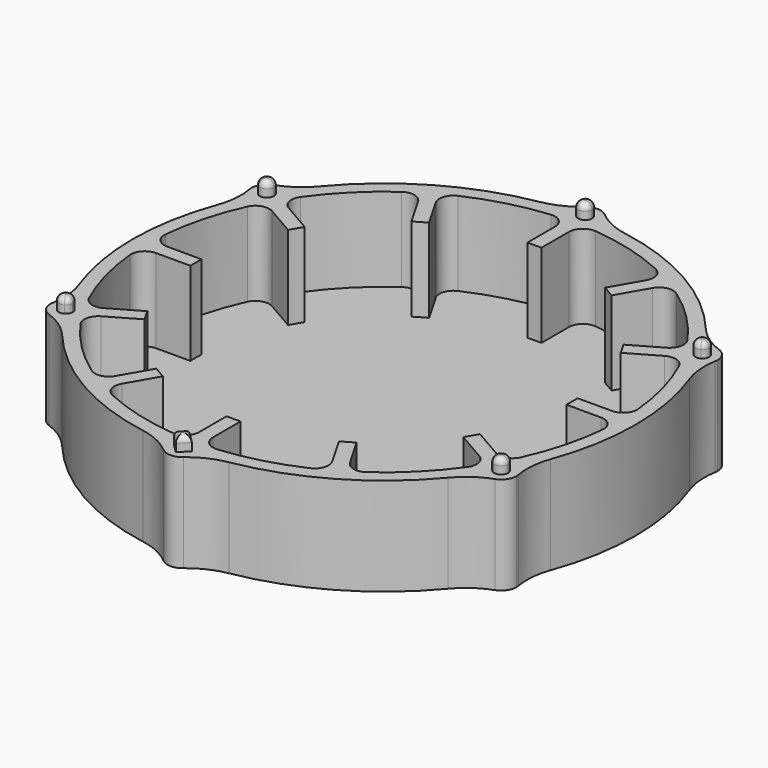
from build123d import *

# Parameters (mm, degrees)
F1_R      = 18
F1_R_2    = 17
F2_DEPTH  = 7
F3_DEPTH  = 7
F4_DEPTH  = 1
F6_DEPTH  = 7
F7_R      = 1
F8_R      = 5
F9_DEPTH  = 8
F10_R     = 0.44999
F11_DEPTH = 1.8


# Not quite as in the source:
# - a fillet or chamfer is up to 0.001 mm smaller than in the source, because OpenCascade refuses the exact size


with BuildPart() as f2:
    # F1 (on Top) → F2 (new body)
    with BuildSketch(Plane.XY):
        Circle(F1_R)
        Circle(F1_R_2, mode=Mode.SUBTRACT)
    extrude(amount=F2_DEPTH)

    # F0 (on Top) → F3 (join)
    with BuildSketch(Plane.XY):
        with BuildLine():
            Line((-11.4073228059, 7.1633711619), (-14.4660626528, 8.9293354359))
            ThreePointArc((-14.4660626528, 8.9293354359), (-14.7224318643, 8.5), (-14.9660626528, 8.0633100321))
            Line((-14.9660626528, 8.0633100321), (-11.9073228059, 6.2973457581))
            ThreePointArc((-11.9073228059, 6.2973457581), (-11.665362189, 6.735), (-11.4073228059, 7.1633711619))
        make_face()
        with BuildLine():
            Line((7.1633711619, 11.4073228059), (8.9293354359, 14.4660626528))
            ThreePointArc((8.9293354359, 14.4660626528), (8.5, 14.7224318643), (8.0633100321, 14.9660626528))
            Line((8.0633100321, 14.9660626528), (6.2973457581, 11.9073228059))
            ThreePointArc((6.2973457581, 11.9073228059), (6.735, 11.665362189), (7.1633711619, 11.4073228059))
        make_face()
        with BuildLine():
            ThreePointArc((17, 0), (16.9981612676, 0.2500270431), (16.992645468, 0.5))
            Line((16.992645468, 0.5), (13.46071692, 0.5))
            ThreePointArc((13.46071692, 0.5), (13.46767903, 0.2500430841), (13.47, 0))
            ThreePointArc((13.47, 0), (13.46767903, -0.2500430841), (13.46071692, -0.5))
            Line((13.46071692, -0.5), (16.992645468, -0.5))
            ThreePointArc((16.992645468, -0.5), (16.9981612676, -0.2500270431), (17, 0))
        make_face()
        with BuildLine():
            ThreePointArc((-0.5, -16.992645468), (0, -17), (0.5, -16.992645468))
            Line((0.5, -16.992645468), (0.5, -13.46071692))
            ThreePointArc((0.5, -13.46071692), (0, -13.47), (-0.5, -13.46071692))
            Line((-0.5, -13.46071692), (-0.5, -16.992645468))
        make_face()
        with BuildLine():
            ThreePointArc((-14.9660626528, -8.0633100321), (-14.7224318643, -8.5), (-14.4660626528, -8.9293354359))
            Line((-14.4660626528, -8.9293354359), (-11.4073228059, -7.1633711619))
            ThreePointArc((-11.4073228059, -7.1633711619), (-11.665362189, -6.735), (-11.9073228059, -6.2973457581))
            Line((-11.9073228059, -6.2973457581), (-14.9660626528, -8.0633100321))
        make_face()
        with BuildLine():
            Line((-6.2973457581, 11.9073228059), (-8.0633100321, 14.9660626528))
            ThreePointArc((-8.0633100321, 14.9660626528), (-8.5, 14.7224318643), (-8.9293354359, 14.4660626528))
            Line((-8.9293354359, 14.4660626528), (-7.1633711619, 11.4073228059))
            ThreePointArc((-7.1633711619, 11.4073228059), (-6.735, 11.665362189), (-6.2973457581, 11.9073228059))
        make_face()
        with BuildLine():
            Line((0.5, 13.46071692), (0.5, 16.992645468))
            ThreePointArc((0.5, 16.992645468), (0, 17), (-0.5, 16.992645468))
            Line((-0.5, 16.992645468), (-0.5, 13.46071692))
            ThreePointArc((-0.5, 13.46071692), (0, 13.47), (0.5, 13.46071692))
        make_face()
        with BuildLine():
            Line((11.9073228059, 6.2973457581), (14.9660626528, 8.0633100321))
            ThreePointArc((14.9660626528, 8.0633100321), (14.7224318643, 8.5), (14.4660626528, 8.9293354359))
            Line((14.4660626528, 8.9293354359), (11.4073228059, 7.1633711619))
            ThreePointArc((11.4073228059, 7.1633711619), (11.665362189, 6.735), (11.9073228059, 6.2973457581))
        make_face()
        with BuildLine():
            ThreePointArc((14.4660626528, -8.9293354359), (14.7224318643, -8.5), (14.9660626528, -8.0633100321))
            Line((14.9660626528, -8.0633100321), (11.9073228059, -6.2973457581))
            ThreePointArc((11.9073228059, -6.2973457581), (11.665362189, -6.735), (11.4073228059, -7.1633711619))
            Line((11.4073228059, -7.1633711619), (14.4660626528, -8.9293354359))
        make_face()
        with BuildLine():
            ThreePointArc((8.0633100321, -14.9660626528), (8.5, -14.7224318643), (8.9293354359, -14.4660626528))
            Line((8.9293354359, -14.4660626528), (7.1633711619, -11.4073228059))
            ThreePointArc((7.1633711619, -11.4073228059), (6.735, -11.665362189), (6.2973457581, -11.9073228059))
            Line((6.2973457581, -11.9073228059), (8.0633100321, -14.9660626528))
        make_face()
        with BuildLine():
            ThreePointArc((-8.9293354359, -14.4660626528), (-8.5, -14.7224318643), (-8.0633100321, -14.9660626528))
            Line((-8.0633100321, -14.9660626528), (-6.2973457581, -11.9073228059))
            ThreePointArc((-6.2973457581, -11.9073228059), (-6.735, -11.665362189), (-7.1633711619, -11.4073228059))
            Line((-7.1633711619, -11.4073228059), (-8.9293354359, -14.4660626528))
        make_face()
        with BuildLine():
            Line((-13.46071692, 0.5), (-16.992645468, 0.5))
            ThreePointArc((-16.992645468, 0.5), (-17, 0), (-16.992645468, -0.5))
            Line((-16.992645468, -0.5), (-13.46071692, -0.5))
            ThreePointArc((-13.46071692, -0.5), (-13.47, 0), (-13.46071692, 0.5))
        make_face()
    extrude(amount=F3_DEPTH)

    # F1 (on Top) → F4 (join)
    with BuildSketch(Plane.XY):
        Circle(F1_R)
        Circle(F1_R_2, mode=Mode.SUBTRACT)
        Circle(F1_R_2)
    extrude(amount=F4_DEPTH)

    # F5 (on Top) → F6 (join)
    with BuildSketch(Plane.XY):
        with BuildLine():
            ThreePointArc((-14.4884572681, 9), (-14.6275367743, 9.5353800561), (-15.0096060035, 9.935377578))
            ThreePointArc((-15.0096060035, 9.935377578), (-15.1731450826, 9.6837837802), (-15.3324673166, 9.4294987133))
            ThreePointArc((-15.3324673166, 9.4294987133), (-15.153718855, 9.2469868663), (-15.0884572681, 9))
            ThreePointArc((-15.0884572681, 9), (-15.3354561915, 8.5687338928), (-15.832419089, 8.5635568422))
            ThreePointArc((-15.832419089, 8.5635568422), (-15.9729752997, 8.2984372068), (-16.1090923805, 8.0310113108))
            ThreePointArc((-16.1090923805, 8.0310113108), (-15.0239657375, 8.0558870238), (-14.4884572681, 9))
        make_face()
        with BuildLine():
            ThreePointArc((-15.3324673166, 9.4294987133), (-15.1731450826, 9.6837837802), (-15.0096060035, 9.935377578))
            ThreePointArc((-15.0096060035, 9.935377578), (-16.5410852123, 9.55), (-16.1090923805, 8.0310113108))
            ThreePointArc((-16.1090923805, 8.0310113108), (-15.9729752997, 8.2984372068), (-15.832419089, 8.5635568422))
            ThreePointArc((-15.832419089, 8.5635568422), (-16.02146997, 9.25), (-15.3324673166, 9.4294987133))
        make_face()
        with BuildLine():
            ThreePointArc((-1.099486377, 17.9663888889), (0, 16.9), (1.099486377, 17.9663888889))
            ThreePointArc((1.099486377, 17.9663888889), (0.7998302171, 17.982220987), (0.4999517724, 17.9930555556))
            ThreePointArc((0.4999517724, 17.9930555556), (0, 17.5), (-0.4999517724, 17.9930555556))
            ThreePointArc((-0.4999517724, 17.9930555556), (-0.7998302171, 17.982220987), (-1.099486377, 17.9663888889))
        make_face()
        with BuildLine():
            ThreePointArc((0.4999517724, 17.9930555556), (0.7998302171, 17.982220987), (1.099486377, 17.9663888889))
            ThreePointArc((1.099486377, 17.9663888889), (1.0998715868, 17.9831924823), (1.1, 18))
            ThreePointArc((1.1, 18), (-0.0168075177, 19.0998715868), (-1.099486377, 17.9663888889))
            ThreePointArc((-1.099486377, 17.9663888889), (-0.7998302171, 17.982220987), (-0.4999517724, 17.9930555556))
            ThreePointArc((-0.4999517724, 17.9930555556), (-0.003472306, 18.4999879429), (0.5, 18))
            ThreePointArc((0.5, 18), (0.4999879429, 17.996527694), (0.4999517724, 17.9930555556))
        make_face()
        with BuildLine():
            ThreePointArc((15.832419089, 8.5635568422), (15.9729752997, 8.2984372068), (16.1090923805, 8.0310113108))
            ThreePointArc((16.1090923805, 8.0310113108), (16.5325702443, 8.4355084694), (16.6884572681, 9))
            ThreePointArc((16.6884572681, 9), (16.1238373242, 9.9609204939), (15.0096060035, 9.935377578))
            ThreePointArc((15.0096060035, 9.935377578), (15.1731450826, 9.6837837802), (15.3324673166, 9.4294987133))
            ThreePointArc((15.3324673166, 9.4294987133), (15.8354441344, 9.4347384132), (16.0884572681, 9))
            ThreePointArc((16.0884572681, 9), (16.0197233753, 8.7469989234), (15.832419089, 8.5635568422))
        make_face()
        with BuildLine():
            ThreePointArc((15.0096060035, 9.935377578), (14.635829324, 8.45), (16.1090923805, 8.0310113108))
            ThreePointArc((16.1090923805, 8.0310113108), (15.9729752997, 8.2984372068), (15.832419089, 8.5635568422))
            ThreePointArc((15.832419089, 8.5635568422), (15.1554445662, 8.75), (15.3324673166, 9.4294987133))
            ThreePointArc((15.3324673166, 9.4294987133), (15.1731450826, 9.6837837802), (15.0096060035, 9.935377578))
        make_face()
        with BuildLine():
            ThreePointArc((-15.3324673166, -9.4294987133), (-15.1731450826, -9.6837837802), (-15.0096060035, -9.935377578))
            ThreePointArc((-15.0096060035, -9.935377578), (-14.6275367743, -9.5353800561), (-14.4884572681, -9))
            ThreePointArc((-14.4884572681, -9), (-15.0239657375, -8.0558870238), (-16.1090923805, -8.0310113108))
            ThreePointArc((-16.1090923805, -8.0310113108), (-15.9729752997, -8.2984372068), (-15.832419089, -8.5635568422))
            ThreePointArc((-15.832419089, -8.5635568422), (-15.3354561915, -8.5687338928), (-15.0884572681, -9))
            ThreePointArc((-15.0884572681, -9), (-15.153718855, -9.2469868663), (-15.3324673166, -9.4294987133))
        make_face()
        with BuildLine():
            ThreePointArc((-16.1090923805, -8.0310113108), (-16.5410852123, -9.55), (-15.0096060035, -9.935377578))
            ThreePointArc((-15.0096060035, -9.935377578), (-15.1731450826, -9.6837837802), (-15.3324673166, -9.4294987133))
            ThreePointArc((-15.3324673166, -9.4294987133), (-16.02146997, -9.25), (-15.832419089, -8.5635568422))
            ThreePointArc((-15.832419089, -8.5635568422), (-15.9729752997, -8.2984372068), (-16.1090923805, -8.0310113108))
        make_face()
        with BuildLine():
            ThreePointArc((0.6255239257, -17.9891278226), (0.8625800837, -17.9793202207), (1.099486377, -17.9663888889))
            ThreePointArc((1.099486377, -17.9663888889), (0, -16.9), (-1.099486377, -17.9663888889))
            ThreePointArc((-1.099486377, -17.9663888889), (-0.8625800837, -17.9793202207), (-0.6255239257, -17.9891278226))
            Line((-0.6255239257, -17.9891278226), (0, -17.3636038969))
            Line((0, -17.3636038969), (0.6255239257, -17.9891278226))
        make_face()
        with BuildLine():
            ThreePointArc((1.1, -18), (1.0998715868, -17.9831924823), (1.099486377, -17.9663888889))
            ThreePointArc((1.099486377, -17.9663888889), (0.8625800837, -17.9793202207), (0.6255239257, -17.9891278226))
            Line((0.6255239257, -17.9891278226), (0.6363961031, -18))
            Line((0.6363961031, -18), (0, -18.6363961031))
            Line((0, -18.6363961031), (-0.6363961031, -18))
            Line((-0.6363961031, -18), (-0.6255239257, -17.9891278226))
            ThreePointArc((-0.6255239257, -17.9891278226), (-0.8625800837, -17.9793202207), (-1.099486377, -17.9663888889))
            ThreePointArc((-1.099486377, -17.9663888889), (-0.0168075177, -19.0998715868), (1.1, -18))
        make_face()
        with BuildLine():
            ThreePointArc((16.6884572681, -9), (16.5325702443, -8.4355084694), (16.1090923805, -8.0310113108))
            ThreePointArc((16.1090923805, -8.0310113108), (15.9729752997, -8.2984372068), (15.832419089, -8.5635568422))
            ThreePointArc((15.832419089, -8.5635568422), (16.0197233753, -8.7469989234), (16.0884572681, -9))
            ThreePointArc((16.0884572681, -9), (15.8354441344, -9.4347384132), (15.3324673166, -9.4294987133))
            ThreePointArc((15.3324673166, -9.4294987133), (15.1731450826, -9.6837837802), (15.0096060035, -9.935377578))
            ThreePointArc((15.0096060035, -9.935377578), (16.1238373242, -9.9609204939), (16.6884572681, -9))
        make_face()
        with BuildLine():
            ThreePointArc((15.832419089, -8.5635568422), (15.9729752997, -8.2984372068), (16.1090923805, -8.0310113108))
            ThreePointArc((16.1090923805, -8.0310113108), (14.635829324, -8.45), (15.0096060035, -9.935377578))
            ThreePointArc((15.0096060035, -9.935377578), (15.1731450826, -9.6837837802), (15.3324673166, -9.4294987133))
            ThreePointArc((15.3324673166, -9.4294987133), (15.1554445662, -8.75), (15.832419089, -8.5635568422))
        make_face()
        with BuildLine():
            ThreePointArc((-15.0884572681, 9), (-15.153718855, 9.2469868663), (-15.3324673166, 9.4294987133))
            ThreePointArc((-15.3324673166, 9.4294987133), (-15.5884572681, 9), (-15.832419089, 8.5635568422))
            ThreePointArc((-15.832419089, 8.5635568422), (-15.3354561915, 8.5687338928), (-15.0884572681, 9))
        make_face()
        with BuildLine():
            ThreePointArc((-15.832419089, 8.5635568422), (-15.5884572681, 9), (-15.3324673166, 9.4294987133))
            ThreePointArc((-15.3324673166, 9.4294987133), (-16.02146997, 9.25), (-15.832419089, 8.5635568422))
        make_face()
        with BuildLine():
            ThreePointArc((-0.4999517724, 17.9930555556), (0, 18), (0.4999517724, 17.9930555556))
            ThreePointArc((0.4999517724, 17.9930555556), (0.4999879429, 17.996527694), (0.5, 18))
            ThreePointArc((0.5, 18), (-0.003472306, 18.4999879429), (-0.4999517724, 17.9930555556))
        make_face()
        with BuildLine():
            ThreePointArc((-0.4999517724, 17.9930555556), (0, 17.5), (0.4999517724, 17.9930555556))
            ThreePointArc((0.4999517724, 17.9930555556), (0, 18), (-0.4999517724, 17.9930555556))
        make_face()
        with BuildLine():
            ThreePointArc((15.3324673166, 9.4294987133), (15.5884572681, 9), (15.832419089, 8.5635568422))
            ThreePointArc((15.832419089, 8.5635568422), (16.0197233753, 8.7469989234), (16.0884572681, 9))
            ThreePointArc((16.0884572681, 9), (15.8354441344, 9.4347384132), (15.3324673166, 9.4294987133))
        make_face()
        with BuildLine():
            ThreePointArc((15.3324673166, 9.4294987133), (15.1554445662, 8.75), (15.832419089, 8.5635568422))
            ThreePointArc((15.832419089, 8.5635568422), (15.5884572681, 9), (15.3324673166, 9.4294987133))
        make_face()
        with BuildLine():
            ThreePointArc((16.0884572681, -9), (16.0197233753, -8.7469989234), (15.832419089, -8.5635568422))
            ThreePointArc((15.832419089, -8.5635568422), (15.5884572681, -9), (15.3324673166, -9.4294987133))
            ThreePointArc((15.3324673166, -9.4294987133), (15.8354441344, -9.4347384132), (16.0884572681, -9))
        make_face()
        with BuildLine():
            ThreePointArc((15.3324673166, -9.4294987133), (15.5884572681, -9), (15.832419089, -8.5635568422))
            ThreePointArc((15.832419089, -8.5635568422), (15.1554445662, -8.75), (15.3324673166, -9.4294987133))
        make_face()
        with BuildLine():
            Line((0.6363961031, -18), (0.6255239257, -17.9891278226))
            ThreePointArc((0.6255239257, -17.9891278226), (0, -18), (-0.6255239257, -17.9891278226))
            Line((-0.6255239257, -17.9891278226), (-0.6363961031, -18))
            Line((-0.6363961031, -18), (0, -18.6363961031))
            Line((0, -18.6363961031), (0.6363961031, -18))
        make_face()
        with BuildLine():
            ThreePointArc((-15.832419089, -8.5635568422), (-16.02146997, -9.25), (-15.3324673166, -9.4294987133))
            ThreePointArc((-15.3324673166, -9.4294987133), (-15.5884572681, -9), (-15.832419089, -8.5635568422))
        make_face()
        with BuildLine():
            ThreePointArc((-15.832419089, -8.5635568422), (-15.5884572681, -9), (-15.3324673166, -9.4294987133))
            ThreePointArc((-15.3324673166, -9.4294987133), (-15.153718855, -9.2469868663), (-15.0884572681, -9))
            ThreePointArc((-15.0884572681, -9), (-15.3354561915, -8.5687338928), (-15.832419089, -8.5635568422))
        make_face()
        with BuildLine():
            ThreePointArc((-0.6255239257, -17.9891278226), (0, -18), (0.6255239257, -17.9891278226))
            Line((0.6255239257, -17.9891278226), (0, -17.3636038969))
            Line((0, -17.3636038969), (-0.6255239257, -17.9891278226))
        make_face()
    extrude(amount=F6_DEPTH)

    # F7
    f7_edges = [f2.edges().sort_by_distance(p)[0] for p in [
        (0.5, -16.992645, 4),
        (-8.929335, -14.466063, 4),
        (-14.966063, -8.06331, 4),
        (-16.992645, 0.5, 4),
        (8.929335, -14.466063, 4),
        (14.966063, -8.06331, 4),
        (-0.5, 16.992645, 4),
        (8.06331, 14.966063, 4),
        (14.466063, 8.929335, 4),
        (16.992645, -0.5, 4),
        (-14.966063, 8.06331, 4),
        (-16.992645, -0.5, 4),
        (-8.929335, 14.466063, 4),
        (0.5, 16.992645, 4),
        (-14.466063, 8.929335, 4),
        (-8.06331, 14.966063, 4),
        (-14.466063, -8.929335, 4),
        (-8.06331, -14.966063, 4),
        (14.966063, 8.06331, 4),
        (8.929335, 14.466063, 4),
        (-0.5, -16.992645, 4),
        (8.06331, -14.966063, 4),
        (14.466063, -8.929335, 4),
        (16.992645, 0.5, 4),
    ]]
    fillet(f7_edges, radius=F7_R)

    # F8 (call 1 of 12: OpenCascade refuses the feature's edges together)
    f8_edges = [f2.edges().sort_by_distance(p)[0] for p in [
        (-16.109092, 8.031011, 3.5),
    ]]
    fillet(f8_edges, radius=F8_R)

    # F8#2 (call 2 of 12)
    f8_2_edges = [f2.edges().sort_by_distance(p)[0] for p in [
        (-15.009606, 9.935378, 3.5),
    ]]
    fillet(f8_2_edges, radius=F8_R)

    # F8#3 (call 3 of 12)
    f8_3_edges = [f2.edges().sort_by_distance(p)[0] for p in [
        (-1.099486, 17.966389, 3.5),
    ]]
    fillet(f8_3_edges, radius=F8_R)

    # F8#4 (call 4 of 12)
    f8_4_edges = [f2.edges().sort_by_distance(p)[0] for p in [
        (1.099486, 17.966389, 3.5),
    ]]
    fillet(f8_4_edges, radius=F8_R)

    # F8#5 (call 5 of 12)
    f8_5_edges = [f2.edges().sort_by_distance(p)[0] for p in [
        (-15.009606, -9.935378, 3.5),
    ]]
    fillet(f8_5_edges, radius=F8_R)

    # F8#6 (call 6 of 12)
    f8_6_edges = [f2.edges().sort_by_distance(p)[0] for p in [
        (-16.109092, -8.031011, 3.5),
    ]]
    fillet(f8_6_edges, radius=F8_R)

    # F8#7 (call 7 of 12)
    f8_7_edges = [f2.edges().sort_by_distance(p)[0] for p in [
        (1.099486, -17.966389, 3.5),
    ]]
    fillet(f8_7_edges, radius=F8_R)

    # F8#8 (call 8 of 12)
    f8_8_edges = [f2.edges().sort_by_distance(p)[0] for p in [
        (-1.099486, -17.966389, 3.5),
    ]]
    fillet(f8_8_edges, radius=F8_R)

    # F8#10 (call 9 of 12)
    f8_10_edges = [f2.edges().sort_by_distance(p)[0] for p in [
        (15.009606, -9.935378, 3.5),
    ]]
    fillet(f8_10_edges, radius=F8_R)

    # F8#11 (call 10 of 12)
    f8_11_edges = [f2.edges().sort_by_distance(p)[0] for p in [
        (16.109092, 8.031011, 3.5),
    ]]
    fillet(f8_11_edges, radius=F8_R)

    # F8#12 (call 11 of 12)
    f8_12_edges = [f2.edges().sort_by_distance(p)[0] for p in [
        (15.009606, 9.935378, 3.5),
    ]]
    fillet(f8_12_edges, radius=F8_R)

    # F8#9 (call 12 of 12)
    f8_9_edges = [f2.edges().sort_by_distance(p)[0] for p in [
        (16.109092, -8.031011, 3.5),
    ]]
    fillet(f8_9_edges, radius=F8_R)

    # F5 (on Top) → F9 (join)
    with BuildSketch(Plane.XY):
        with BuildLine():
            ThreePointArc((-15.832419089, 8.5635568422), (-15.5884572681, 9), (-15.3324673166, 9.4294987133))
            ThreePointArc((-15.3324673166, 9.4294987133), (-16.02146997, 9.25), (-15.832419089, 8.5635568422))
        make_face()
        with BuildLine():
            ThreePointArc((-15.0884572681, 9), (-15.153718855, 9.2469868663), (-15.3324673166, 9.4294987133))
            ThreePointArc((-15.3324673166, 9.4294987133), (-15.5884572681, 9), (-15.832419089, 8.5635568422))
            ThreePointArc((-15.832419089, 8.5635568422), (-15.3354561915, 8.5687338928), (-15.0884572681, 9))
        make_face()
        with BuildLine():
            ThreePointArc((-0.4999517724, 17.9930555556), (0, 18), (0.4999517724, 17.9930555556))
            ThreePointArc((0.4999517724, 17.9930555556), (0.4999879429, 17.996527694), (0.5, 18))
            ThreePointArc((0.5, 18), (-0.003472306, 18.4999879429), (-0.4999517724, 17.9930555556))
        make_face()
        with BuildLine():
            ThreePointArc((-0.4999517724, 17.9930555556), (0, 17.5), (0.4999517724, 17.9930555556))
            ThreePointArc((0.4999517724, 17.9930555556), (0, 18), (-0.4999517724, 17.9930555556))
        make_face()
        with BuildLine():
            ThreePointArc((15.3324673166, 9.4294987133), (15.1554445662, 8.75), (15.832419089, 8.5635568422))
            ThreePointArc((15.832419089, 8.5635568422), (15.5884572681, 9), (15.3324673166, 9.4294987133))
        make_face()
        with BuildLine():
            ThreePointArc((15.3324673166, 9.4294987133), (15.5884572681, 9), (15.832419089, 8.5635568422))
            ThreePointArc((15.832419089, 8.5635568422), (16.0197233753, 8.7469989234), (16.0884572681, 9))
            ThreePointArc((16.0884572681, 9), (15.8354441344, 9.4347384132), (15.3324673166, 9.4294987133))
        make_face()
        with BuildLine():
            ThreePointArc((15.3324673166, -9.4294987133), (15.5884572681, -9), (15.832419089, -8.5635568422))
            ThreePointArc((15.832419089, -8.5635568422), (15.1554445662, -8.75), (15.3324673166, -9.4294987133))
        make_face()
        with BuildLine():
            ThreePointArc((16.0884572681, -9), (16.0197233753, -8.7469989234), (15.832419089, -8.5635568422))
            ThreePointArc((15.832419089, -8.5635568422), (15.5884572681, -9), (15.3324673166, -9.4294987133))
            ThreePointArc((15.3324673166, -9.4294987133), (15.8354441344, -9.4347384132), (16.0884572681, -9))
        make_face()
        with BuildLine():
            Line((0.6363961031, -18), (0.6255239257, -17.9891278226))
            ThreePointArc((0.6255239257, -17.9891278226), (0, -18), (-0.6255239257, -17.9891278226))
            Line((-0.6255239257, -17.9891278226), (-0.6363961031, -18))
            Line((-0.6363961031, -18), (0, -18.6363961031))
            Line((0, -18.6363961031), (0.6363961031, -18))
        make_face()
        with BuildLine():
            ThreePointArc((-0.6255239257, -17.9891278226), (0, -18), (0.6255239257, -17.9891278226))
            Line((0.6255239257, -17.9891278226), (0, -17.3636038969))
            Line((0, -17.3636038969), (-0.6255239257, -17.9891278226))
        make_face()
        with BuildLine():
            ThreePointArc((-15.832419089, -8.5635568422), (-16.02146997, -9.25), (-15.3324673166, -9.4294987133))
            ThreePointArc((-15.3324673166, -9.4294987133), (-15.5884572681, -9), (-15.832419089, -8.5635568422))
        make_face()
        with BuildLine():
            ThreePointArc((-15.832419089, -8.5635568422), (-15.5884572681, -9), (-15.3324673166, -9.4294987133))
            ThreePointArc((-15.3324673166, -9.4294987133), (-15.153718855, -9.2469868663), (-15.0884572681, -9))
            ThreePointArc((-15.0884572681, -9), (-15.3354561915, -8.5687338928), (-15.832419089, -8.5635568422))
        make_face()
    extrude(amount=F9_DEPTH)

    # F10 (radius 0.45 in the source; OpenCascade refuses exactly that, so slightly less here)
    f10_edges = [f2.edges().sort_by_distance(p)[0] for p in [
        (-15.844447, -8.570501, 8),
        (-15.344495, 9.436443, 8),
        (0.499952, 18.006944, 8),
        (15.344495, 9.436443, 8),
        (15.844447, -8.570501, 8),
        (0.318198, -17.681802, 8),
        (-0.318198, -18.318198, 8),
        (0.318198, -18.318198, 8),
        (-0.318198, -17.681802, 8),
    ]]
    fillet(f10_edges, radius=F10_R)

    # F5 (on Top) → F11 (cut)
    with BuildSketch(Plane.XY):
        with BuildLine():
            ThreePointArc((-15.832419089, -8.5635568422), (-16.02146997, -9.25), (-15.3324673166, -9.4294987133))
            ThreePointArc((-15.3324673166, -9.4294987133), (-15.5884572681, -9), (-15.832419089, -8.5635568422))
        make_face()
        with BuildLine():
            ThreePointArc((-15.832419089, -8.5635568422), (-15.5884572681, -9), (-15.3324673166, -9.4294987133))
            ThreePointArc((-15.3324673166, -9.4294987133), (-15.153718855, -9.2469868663), (-15.0884572681, -9))
            ThreePointArc((-15.0884572681, -9), (-15.3354561915, -8.5687338928), (-15.832419089, -8.5635568422))
        make_face()
        with BuildLine():
            Line((0.6363961031, -18), (0.6255239257, -17.9891278226))
            ThreePointArc((0.6255239257, -17.9891278226), (0, -18), (-0.6255239257, -17.9891278226))
            Line((-0.6255239257, -17.9891278226), (-0.6363961031, -18))
            Line((-0.6363961031, -18), (0, -18.6363961031))
            Line((0, -18.6363961031), (0.6363961031, -18))
        make_face()
        with BuildLine():
            ThreePointArc((-0.6255239257, -17.9891278226), (0, -18), (0.6255239257, -17.9891278226))
            Line((0.6255239257, -17.9891278226), (0, -17.3636038969))
            Line((0, -17.3636038969), (-0.6255239257, -17.9891278226))
        make_face()
        with BuildLine():
            ThreePointArc((15.3324673166, -9.4294987133), (15.5884572681, -9), (15.832419089, -8.5635568422))
            ThreePointArc((15.832419089, -8.5635568422), (15.1554445662, -8.75), (15.3324673166, -9.4294987133))
        make_face()
        with BuildLine():
            ThreePointArc((16.0884572681, -9), (16.0197233753, -8.7469989234), (15.832419089, -8.5635568422))
            ThreePointArc((15.832419089, -8.5635568422), (15.5884572681, -9), (15.3324673166, -9.4294987133))
            ThreePointArc((15.3324673166, -9.4294987133), (15.8354441344, -9.4347384132), (16.0884572681, -9))
        make_face()
        with BuildLine():
            ThreePointArc((15.3324673166, 9.4294987133), (15.1554445662, 8.75), (15.832419089, 8.5635568422))
            ThreePointArc((15.832419089, 8.5635568422), (15.5884572681, 9), (15.3324673166, 9.4294987133))
        make_face()
        with BuildLine():
            ThreePointArc((15.3324673166, 9.4294987133), (15.5884572681, 9), (15.832419089, 8.5635568422))
            ThreePointArc((15.832419089, 8.5635568422), (16.0197233753, 8.7469989234), (16.0884572681, 9))
            ThreePointArc((16.0884572681, 9), (15.8354441344, 9.4347384132), (15.3324673166, 9.4294987133))
        make_face()
        with BuildLine():
            ThreePointArc((-0.4999517724, 17.9930555556), (0, 17.5), (0.4999517724, 17.9930555556))
            ThreePointArc((0.4999517724, 17.9930555556), (0, 18), (-0.4999517724, 17.9930555556))
        make_face()
        with BuildLine():
            ThreePointArc((-0.4999517724, 17.9930555556), (0, 18), (0.4999517724, 17.9930555556))
            ThreePointArc((0.4999517724, 17.9930555556), (0.4999879429, 17.996527694), (0.5, 18))
            ThreePointArc((0.5, 18), (-0.003472306, 18.4999879429), (-0.4999517724, 17.9930555556))
        make_face()
        with BuildLine():
            ThreePointArc((-15.832419089, 8.5635568422), (-15.5884572681, 9), (-15.3324673166, 9.4294987133))
            ThreePointArc((-15.3324673166, 9.4294987133), (-16.02146997, 9.25), (-15.832419089, 8.5635568422))
        make_face()
        with BuildLine():
            ThreePointArc((-15.0884572681, 9), (-15.153718855, 9.2469868663), (-15.3324673166, 9.4294987133))
            ThreePointArc((-15.3324673166, 9.4294987133), (-15.5884572681, 9), (-15.832419089, 8.5635568422))
            ThreePointArc((-15.832419089, 8.5635568422), (-15.3354561915, 8.5687338928), (-15.0884572681, 9))
        make_face()
    extrude(amount=F11_DEPTH, mode=Mode.SUBTRACT)


solid = f2.part
